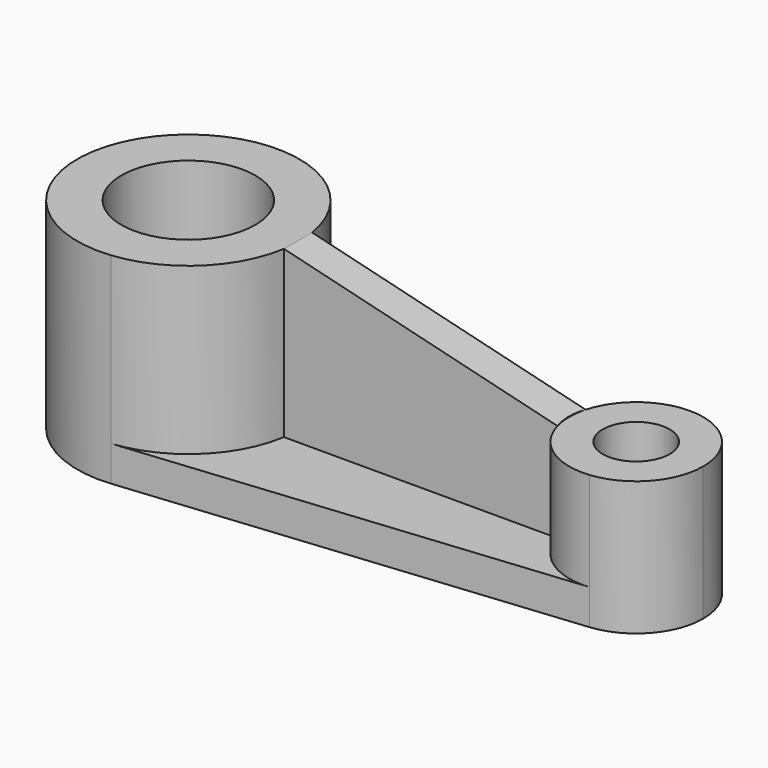
from build123d import *

# Parameters (mm, degrees)
F0_R     = 19
F1_DEPTH = 57
F2_DEPTH = 10
F0_R_2   = 9.5
F3_DEPTH = 38
F5_DEPTH = 57
F7_DEPTH = 36.501


with BuildPart() as f1:
    # F0 (on Top) → F1 (new body)
    with BuildSketch(Plane.XY):
        with BuildLine():
            ThreePointArc((-95.8993569198, 5), (-105.4051754039, 22.9328051198), (-123.8763790613, 31.3447442521))
            ThreePointArc((-123.8763790613, 31.3447442521), (-158.499997838, 0.011670713), (-123.8996062992, -31.3470502424))
            ThreePointArc((-123.8996062992, -31.3470502424), (-105.4136734635, -22.940804403), (-95.8993569198, -5))
            ThreePointArc((-95.8993569198, -5), (-95.5999979536, -2.50796162), (-95.5, 0))
            ThreePointArc((-95.5, 0), (-95.5999979536, 2.50796162), (-95.8993569198, 5))
        make_face()
        with Locations((-127, 0)):
            Circle(F0_R, mode=Mode.SUBTRACT)
    extrude(amount=F1_DEPTH)

    # F0 (on Top) → F2 (join)
    with BuildSketch(Plane.XY):
        with BuildLine():
            Line((-123.8996062992, -31.3470502424), (1.8700787402, -18.9077445907))
            ThreePointArc((1.8700787402, -18.9077445907), (-10.7745572419, -15.6495660081), (-18.3303027798, -5))
            Line((-18.3303027798, -5), (-95.8993569198, -5))
            ThreePointArc((-95.8993569198, -5), (-105.4136734635, -22.940804403), (-123.8996062992, -31.3470502424))
        make_face()
        with BuildLine():
            ThreePointArc((-18.3303027798, 5), (-11.5325625947, 15.0996688705), (0, 19))
            Line((0, 19), (-123.8763790613, 31.3447442521))
            ThreePointArc((-123.8763790613, 31.3447442521), (-105.4051754039, 22.9328051198), (-95.8993569198, 5))
            Line((-95.8993569198, 5), (-18.3303027798, 5))
        make_face()
    extrude(amount=F2_DEPTH)

    # F0 (on Top) → F3 (join)
    with BuildSketch(Plane.XY):
        with BuildLine():
            ThreePointArc((1.8700787402, -18.9077445907), (14.0806870582, -12.7567335932), (19, 0))
            ThreePointArc((19, 0), (13.4350288425, 13.4350288425), (0, 19))
            ThreePointArc((0, 19), (-11.5325625947, 15.0996688705), (-18.3303027798, 5))
            ThreePointArc((-18.3303027798, 5), (-19, 0), (-18.3303027798, -5))
            ThreePointArc((-18.3303027798, -5), (-10.7745572419, -15.6495660081), (1.8700787402, -18.9077445907))
        make_face()
        Circle(F0_R_2, mode=Mode.SUBTRACT)
    extrude(amount=F3_DEPTH)

    # F0 (on Top) → F5 (join)
    with BuildSketch(Plane.XY):
        with BuildLine():
            ThreePointArc((-18.3303027798, -5), (-19, 0), (-18.3303027798, 5))
            Line((-18.3303027798, 5), (-95.8993569198, 5))
            ThreePointArc((-95.8993569198, 5), (-95.5999979536, 2.50796162), (-95.5, 0))
            ThreePointArc((-95.5, 0), (-95.5999979536, -2.50796162), (-95.8993569198, -5))
            Line((-95.8993569198, -5), (-18.3303027798, -5))
        make_face()
    extrude(amount=F5_DEPTH)

    # F6 (on face) → F7 (cut, through all)
    with BuildSketch(Plane.XZ.offset(5)):
        Polygon((-18.3303027798, 57), (-95.8993569198, 57), (-18.3303027798, 38), align=None)
    extrude(amount=-F7_DEPTH, mode=Mode.SUBTRACT)


solid = f1.part
